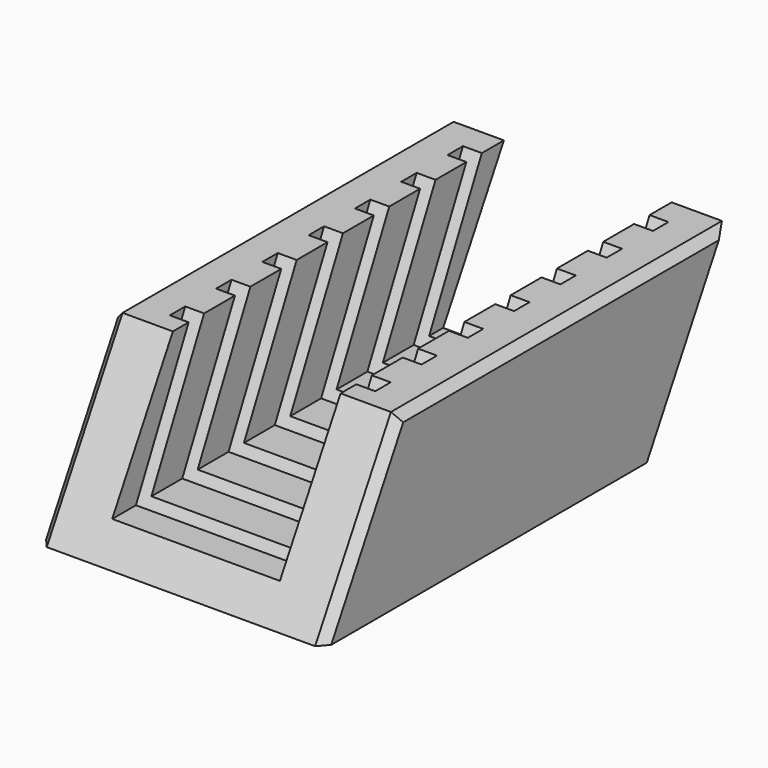
from build123d import *

# Parameters (mm, degrees)
F1_DEPTH = 17
F4_DEPTH = 12.25
F5_W     = 20
F5_H     = 25
F6_DEPTH = 59.5
F7_SIZE  = 1


# Not quite as in the source:
# - a pattern or mirror of a feature is missing from the dataset's text; its kind, count and spacing are read off the source's solid


with BuildPart() as f1:
    # F0 (on Right) → F1 (new body)
    with BuildSketch(Plane.YZ):
        Polygon((23.2368825362, 3.5095077381), (-26.1057236772, 3.5095077381), (-37.4057242716, -16.4904922619), (11.9368819419, -16.4904922619), align=None)
    extrude(amount=F1_DEPTH)

    # F2: F1 across face


with BuildPart() as f1_1:
    add(f1.part)
    add(f1.part.mirror(Plane(origin=(0, -7.0844208677, -6.4904922619), x_dir=(0, 1, 0), z_dir=(-1, 0, 0))))

    # F3 (on Right) → F4 (cut)
    with BuildSketch(Plane.YZ):
        Polygon((-19.8945637886, 6.6848602181), (-22.1945637886, 6.6848602181), (-32.3429037909, -13.9904922619), (-30.0429037909, -13.9904922619), align=None)
        Polygon((-12.9945637886, 6.6848602181), (-15.2945637886, 6.6848602181), (-25.4429037909, -13.9904922619), (-23.1429037909, -13.9904922619), align=None)
        Polygon((-6.0945637886, 6.6848602181), (-8.3945637886, 6.6848602181), (-18.5429037909, -13.9904922619), (-16.2429037909, -13.9904922619), align=None)
        Polygon((0.8054362114, 6.6848602181), (-1.4945637886, 6.6848602181), (-11.6429037909, -13.9904922619), (-9.3429037909, -13.9904922619), align=None)
        Polygon((7.7054362114, 6.6848602181), (5.4054362114, 6.6848602181), (-4.7429037909, -13.9904922619), (-2.4429037909, -13.9904922619), align=None)
        Polygon((14.6054362114, 6.6848602181), (12.3054362114, 6.6848602181), (2.1570962091, -13.9904922619), (4.4570962091, -13.9904922619), align=None)
        Polygon((21.5054362114, 6.6848602181), (19.2054362114, 6.6848602181), (9.0570962091, -13.9904922619), (11.3570962091, -13.9904922619), align=None)
    f4 = extrude(amount=F4_DEPTH, mode=Mode.SUBTRACT)

    # F4_copies: F4 across plane
    add(f4.mirror(Plane(origin=(0, 0, 0), x_dir=(0, 0, -1), z_dir=(-1, 0, 0))), mode=Mode.SUBTRACT)

    # F5 (on Front) → F6 (cut, symmetric)
    with BuildSketch(Plane.XZ):
        Rectangle(F5_W, F5_H)
    extrude(amount=F6_DEPTH, both=True, mode=Mode.SUBTRACT)

    # F7
    f7_edges = [f1_1.edges().sort_by_distance(p)[0] for p in [
        (-17, -1.434421, 3.509508),
        (17, -1.434421, 3.509508),
        (17, -31.755724, -6.490492),
        (17, 17.586882, -6.490492),
        (-17, 17.586882, -6.490492),
        (-17, -31.755724, -6.490492),
    ]]
    chamfer(f7_edges, length=F7_SIZE)


solid = f1_1.part
